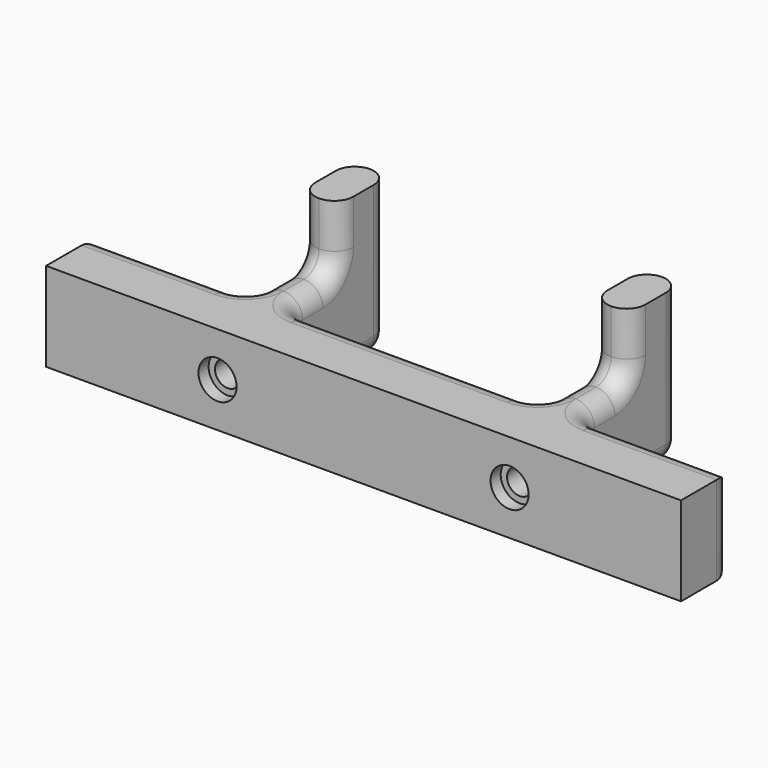
from build123d import *

# Parameters (mm, degrees)
F0_W           = 30
F0_H           = 100
F1_DEPTH       = 70
F2_W           = 30
F2_H           = 50
F3_DEPTH       = 50
F4_F1_R        = 15
F4_F2_R        = 14.9999
F6_D           = 20
F6_DEPTH       = 50
F6_CBORE_D     = 30
F6_CBORE_DEPTH = 10
F6_TIP         = 6.0086061903


# Not quite as in the source:
# - a fillet or chamfer is up to 0.001 mm smaller than in the source, because OpenCascade refuses the exact size


with BuildPart() as f1:
    # F0 (on Top) → F1 (new body)
    with BuildSketch(Plane.XY):
        Polygon((-130, 0), (-250, 0), (-250, -50), (250, -50), (250, 0), (130, 0), (100, 0), (-100, 0), align=None)
        with Locations((-115, 50)):
            Rectangle(F0_W, F0_H)
        with Locations((115, 50)):
            Rectangle(F0_W, F0_H)
    extrude(amount=F1_DEPTH)

    # F2 (on face) → F3 (join)
    with BuildSketch(Plane.XY.offset(70)):
        with Locations((-115, 75)):
            Rectangle(F2_W, F2_H)
        with Locations((115, 75)):
            Rectangle(F2_W, F2_H)
    extrude(amount=F3_DEPTH)

    # F4: fillet of radius 15 on 24 edges, made by hand

    # F4_f1
    f4_f1_edges = [f1.edges().sort_by_distance(p)[0] for p in [
        (-115, 50, 70),
        (115, 50, 70),
        (100, 0, 35),
        (-130, 0, 35),
        (-100, 0, 35),
        (130, 0, 35),
    ]]
    fillet(f4_f1_edges, radius=F4_F1_R)

    # F4_f2 (radius 15 in the source; OpenCascade refuses exactly that, so slightly less here)
    f4_f2_edges = [f1.edges().sort_by_distance(p)[0] for p in [
        (-197.5, 0, 70),
        (115, 100, 0),
        (197.5, 0, 0),
        (197.5, 0, 70),
        (250, 0, 35),
        (130, 100, 60),
        (100, 100, 60),
        (-197.5, 0, 0),
        (-250, 0, 35),
        (-100, 100, 60),
        (-115, 100, 0),
        (-130, 100, 60),
        (0, 0, 70),
        (130, 57.5, 0),
        (100, 57.5, 0),
        (0, 0, 0),
        (-100, 57.5, 0),
        (-130, 57.5, 0),
        (-134.3933982822, 4.3933982822, 0),
        (-95.6066017178, 4.3933982822, 0),
        (95.6066017178, 4.3933982822, 0),
        (134.3933982822, 4.3933982822, 0),
        (95.6066017178, 4.3933982822, 70),
        (-95.6066017178, 4.3933982822, 70),
        (134.3933982822, 4.3933982822, 70),
        (-134.3933982822, 4.3933982822, 70),
    ]]
    fillet(f4_f2_edges, radius=F4_F2_R)

    # F6
    with Locations(Plane.XZ.offset(50)):
        with Locations((-114.9999999844, 35), (115.0000000156, 35)):
            CounterBoreHole(F6_D / 2, F6_CBORE_D / 2, F6_CBORE_DEPTH, depth=F6_DEPTH)
            with Locations((0, 0, -(F6_DEPTH + F6_TIP / 2))):  # 118° drill point
                Cone(0, F6_D / 2, F6_TIP, mode=Mode.SUBTRACT)


solid = f1.part
